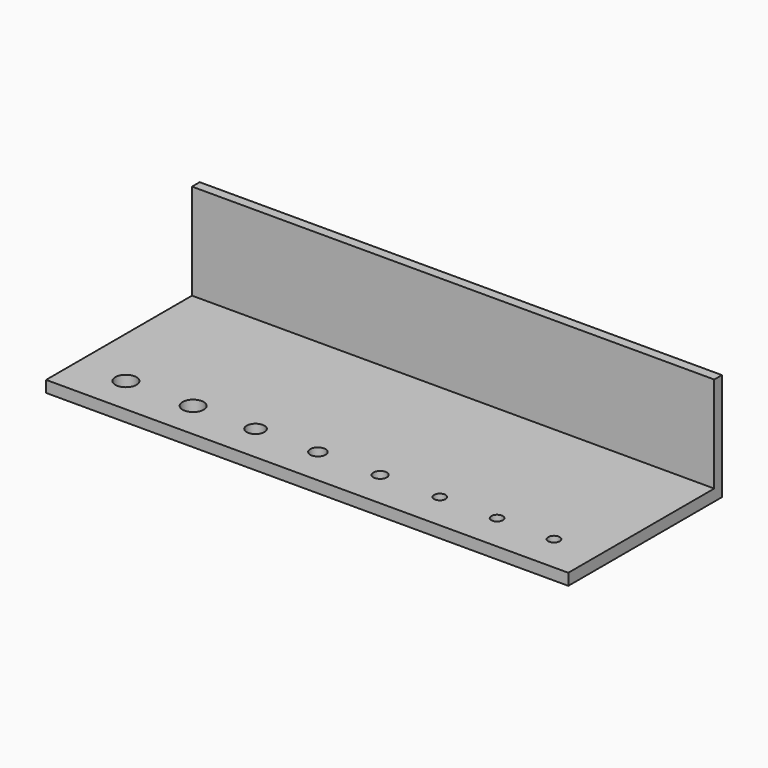
from build123d import *

# Parameters (mm, degrees)
F0_W      = 272
F0_H      = 19.490359351
F0_H_2    = 30.509640649
F1_DEPTH  = 6
F2_D      = 11
F3_D      = 11
F4_D      = 9.2
F5_D      = 8
F6_D      = 7
F7_D      = 6
F8_D      = 6
F9_D      = 6
F10_DEPTH = 50
F11_W     = 272
F11_H     = 5
F12_DEPTH = 50


with BuildPart() as f1:
    # F0 (on Top) → F1 (new body)
    with BuildSketch(Plane.XY):
        with Locations((-83.9492530227, -9.7451796755)):
            Rectangle(F0_W, F0_H)
        with Locations((-83.9492530227, 15.2548203245)):
            Rectangle(F0_W, F0_H_2)
    extrude(amount=-F1_DEPTH)

    # F2 (through all)
    with Locations(Plane.XY):
        with Locations((-193.9492530227, 0)):
            Hole(F2_D / 2)

    # F3 (through all)
    with Locations(Plane.XY):
        with Locations((-158.9492530227, 0)):
            Hole(F3_D / 2)

    # F4 (through all)
    with Locations(Plane.XY):
        with Locations((-126.4492530227, 0)):
            Hole(F4_D / 2)

    # F5 (through all)
    with Locations(Plane.XY):
        with Locations((-93.9492530227, 0)):
            Hole(F5_D / 2)

    # F6 (through all)
    with Locations(Plane.XY):
        with Locations((-61.5492530227, 0)):
            Hole(F6_D / 2)

    # F7 (through all)
    with Locations(Plane.XY):
        with Locations((-30.4492530227, 0)):
            Hole(F7_D / 2)

    # F8 (through all)
    with Locations(Plane.XY):
        with Locations((29.0007469773, 0)):
            Hole(F8_D / 2)

    # F9 (through all)
    with Locations(Plane.XY):
        with Locations((-0.6492530227, 0)):
            Hole(F9_D / 2)

    # F10 (add): a face of the model
    f10_faces = [f1.faces().sort_by_distance(p)[0] for p in [
        (-83.9492530227, 30.509640649, -3),
    ]]
    extrude(f10_faces, amount=F10_DEPTH)

    # F11 (on face) → F12 (join)
    with BuildSketch(Plane.XY):
        with Locations((-83.9492530227, 78.009640649)):
            Rectangle(F11_W, F11_H)
    extrude(amount=F12_DEPTH)


solid = f1.part
